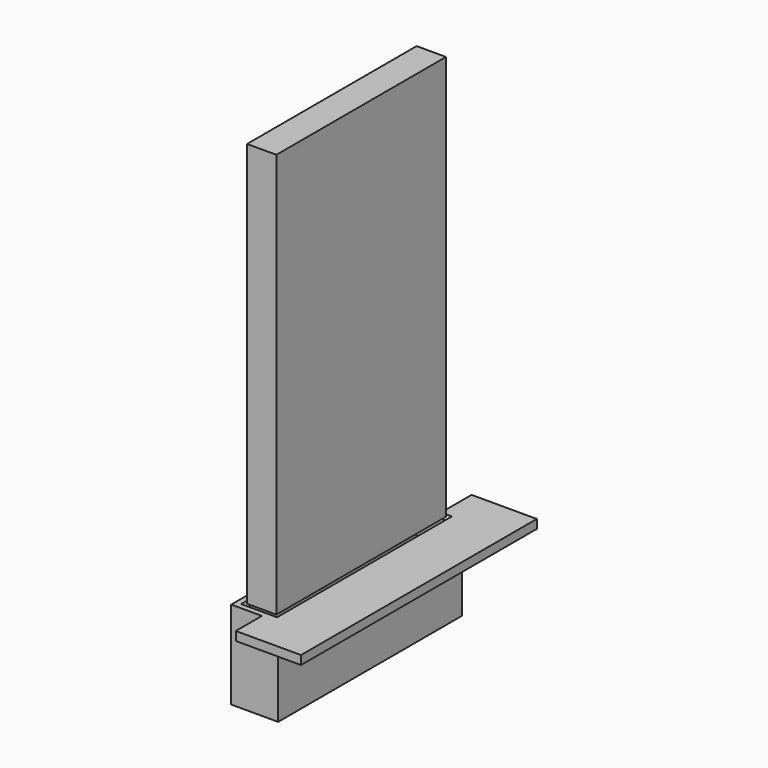
from build123d import *

# Parameters (mm, degrees)
F0_W      = 9
F0_H      = 65
F1_DEPTH  = 124.1524014622
F3_W      = 14.4
F3_H      = 70.4
F3_W_2    = 9
F3_H_2    = 65
F4_DEPTH  = 27
F5_W      = 70.4
F5_H      = 2.7
F6_DEPTH  = 15
F8_DEPTH  = 10
F10_W     = 9
F10_H     = 10
F10_W_2   = 2.7
F11_DEPTH = 4.8
F12_SIZE  = 1


with BuildPart() as f1:
    # F0 (on Top) → F1 (new body)
    with BuildSketch(Plane.XY):
        Rectangle(F0_W, F0_H)
    extrude(amount=F1_DEPTH)


with BuildPart() as f4:
    # F3 (on face) → F4 (new body)
    with BuildSketch(Plane.XY):
        Rectangle(F3_W, F3_H)
        Rectangle(F3_W_2, F3_H_2, mode=Mode.SUBTRACT)
    extrude(amount=-F4_DEPTH)

    # F5 (on face) → F6 (join)
    with BuildSketch(Plane.YZ.offset(7.2)):
        with Locations((0, -1.35)):
            Rectangle(F5_W, F5_H)
    extrude(amount=F6_DEPTH)

    # F7 (on face) → F8 (join)
    with BuildSketch(Plane.XZ.offset(35.2)):
        Polygon((22.2, -2.7), (22.2, 0), (2.2, 0), (2.2, -2.7), (7.2, -2.7), align=None)
    extrude(amount=F8_DEPTH)

    # F9: F4 across plane


with BuildPart() as f4_1:
    add(f4.part)
    add(f4.part.mirror(Plane.XZ))

    # F10 (on face) → F11 (join)
    with BuildSketch(Plane(origin=(0, 0, -27), x_dir=(1, 0, 0), z_dir=(0, 0, -1))):
        Rectangle(F10_W, F10_H)
        with Locations((-5.85, 0)):
            Rectangle(F10_W_2, F10_H)
        with Locations((5.85, 0)):
            Rectangle(F10_W_2, F10_H)
    extrude(amount=-F11_DEPTH)

    # F12
    f12_edges = [f4_1.edges().sort_by_distance(p)[0] for p in [
        (4.5, 0, 0),
        (0, -32.5, 0),
        (-4.5, 0, 0),
        (0, 32.5, 0),
    ]]
    chamfer(f12_edges, length=F12_SIZE)


solid = Compound([f1.part, f4_1.part])
